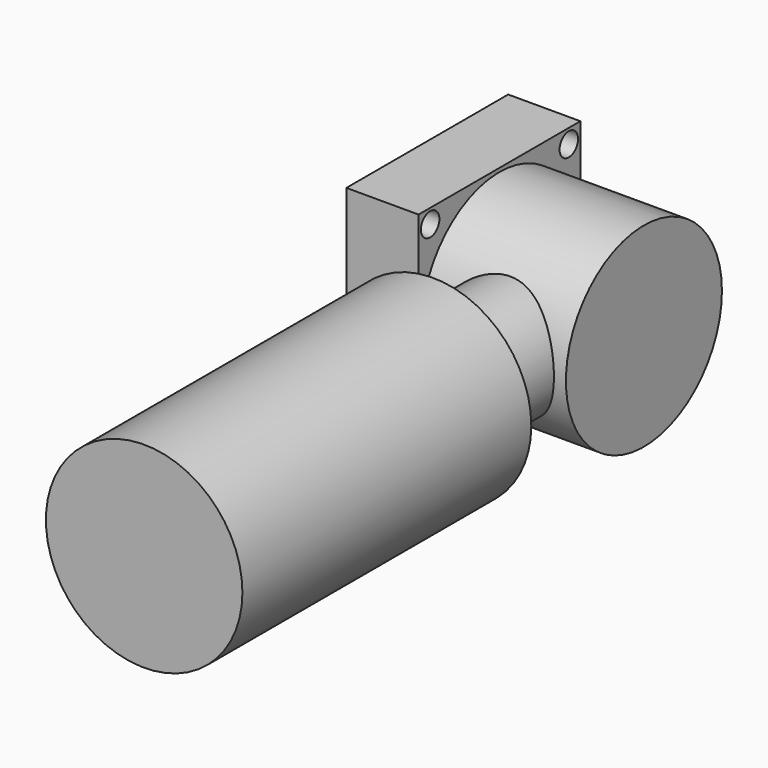
from build123d import *

# Parameters (mm, degrees)
F0_W          = 140
F0_H          = 140
F0_R          = 67.5
F1_DEPTH      = 50
F2_R          = 67.5
F3_DEPTH      = 100
F3_DEPTH_BACK = 25
F4_R          = 41.6737233106
F5_DEPTH      = 120
F6_R          = 68.028235637
F6_R_2        = 41.6737233106
F7_DEPTH      = 250
F8_DEPTH      = 370
F9_R          = 8
F10_DEPTH     = 25


with BuildPart() as f1:
    # F0 (on Right) → F1 (new body)
    with BuildSketch(Plane.YZ):
        Rectangle(F0_W, F0_H)
        Circle(F0_R, mode=Mode.SUBTRACT)
    extrude(amount=-F1_DEPTH)

    # F9 (on face) → F10 (cut, symmetric)
    with BuildSketch(Plane(origin=(-25, 0, 0), x_dir=(0, -1, 0), z_dir=(-1, 0, 0))):
        with Locations((60, 60)):
            Circle(F9_R)
        with Locations((-60, 60)):
            Circle(F9_R)
        with Locations((-60, -60)):
            Circle(F9_R)
        with Locations((60, -60)):
            Circle(F9_R)
    extrude(amount=F10_DEPTH, both=True, mode=Mode.SUBTRACT)


with BuildPart() as f3:
    # F2 (on face) → F3 (new body, two sides)
    with BuildSketch(Plane.YZ) as f3_sk:
        Circle(F2_R)
    extrude(amount=F3_DEPTH)
    extrude(f3_sk.sketch, amount=-F3_DEPTH_BACK)

    # F4 (on Front) → F5 (join)
    with BuildSketch(Plane.XZ):
        with Locations((50, 0)):
            Circle(F4_R)
    extrude(amount=F5_DEPTH)

    # F6 (on face) → F7 (join)
    with BuildSketch(Plane.XZ.offset(120)):
        with Locations((50, 0)):
            Circle(F6_R)
        with Locations((50, 0)):
            Circle(F6_R_2, mode=Mode.SUBTRACT)
    extrude(amount=F7_DEPTH)

    # F4 (on Front) → F8 (join, through all)
    with BuildSketch(Plane.XZ):
        with Locations((50, 0)):
            Circle(F4_R)
    extrude(amount=F8_DEPTH)


solid = Compound([f1.part, f3.part])
